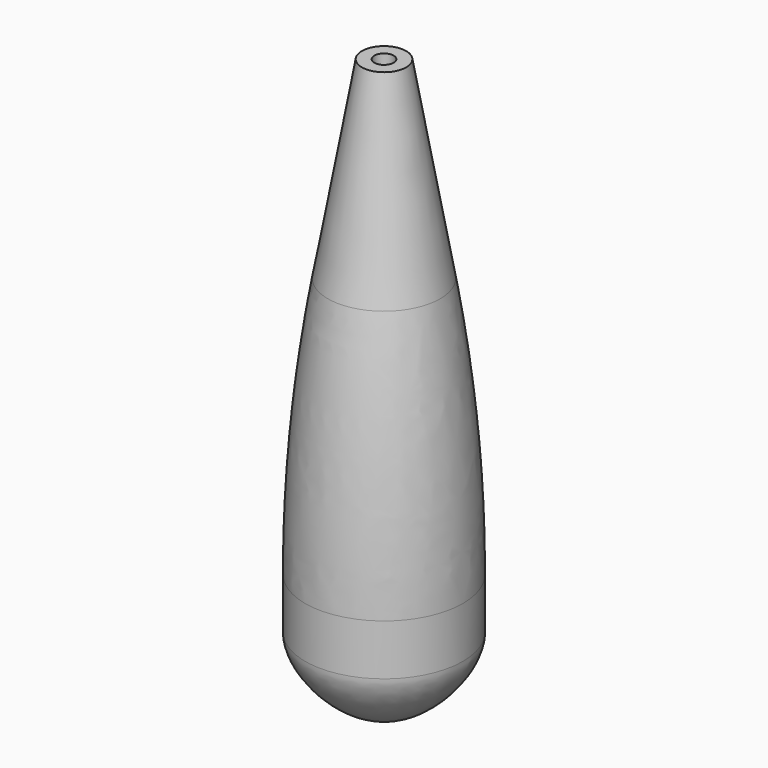
from build123d import *

# Parameters (mm, degrees)
F0_R     = 13.75969411
F1_DEPTH = 100
F3_DEPTH = 100.001
F4_SIZE2 = 56.1456900142
F4_SIZE  = 9.9
F5_R     = 261.7912381488


# Not quite as in the source:
# - a fillet or chamfer that OpenCascade refuses, or shapes differently, is made with other operations: its cross-section is extruded or revolved along the edge and cut away or added


with BuildPart() as f1:
    # F0 (on Top) → F1 (new body)
    with BuildSketch(Plane.XY):
        with Locations((-55.1216676831, -44.3151853979)):
            Circle(F0_R)
    extrude(amount=F1_DEPTH)

    # F2: fillet of radius 12.0710678119 on 1 edges, made by hand

    # F2_s1 → F2_t2 (revolve, cut)
    with BuildSketch(Plane.XZ.offset(44.3151853979)):
        with BuildLine():
            add(Edge.make_bspline(
                [(-41.3619735731, 12.0710678119), (-41.3619735731, 0), (-53.433041385, 0)],
                knots=[0, 0, 0, 1, 1, 1], degree=2, weights=[1, 0.4285714286, 1]))
            Line((-53.433041385, 0), (-41.3619735731, 0))
            Line((-41.3619735731, 0), (-41.3619735731, 12.0710678119))
        make_face()
    revolve(axis=Axis((-55.1216676831, -44.3151853979, 0), (0, 0, 1)), mode=Mode.SUBTRACT)

    # F3 (cut, through all): a face of the model
    f3_faces = [f1.faces().sort_by_distance(p)[0] for p in [
        (-55.1216676831, -44.3151853979, 0),
    ]]
    extrude(f3_faces, amount=-F3_DEPTH, mode=Mode.SUBTRACT)

    # F4
    f4_edges = [f1.edges().sort_by_distance(p)[0] for p in [
        (-68.881362, -44.315185, 100),
    ]]
    f4_side = f1.faces().sort_by_distance((-68.492179, -44.315185, 100))[0]
    chamfer(f4_edges, length=F4_SIZE, length2=F4_SIZE2, reference=f4_side)

    # F5
    f5_edges = [f1.edges().sort_by_distance(p)[0] for p in [
        (-68.881362, -44.315185, 43.85431),
    ]]
    fillet(f5_edges, radius=F5_R)


solid = f1.part
